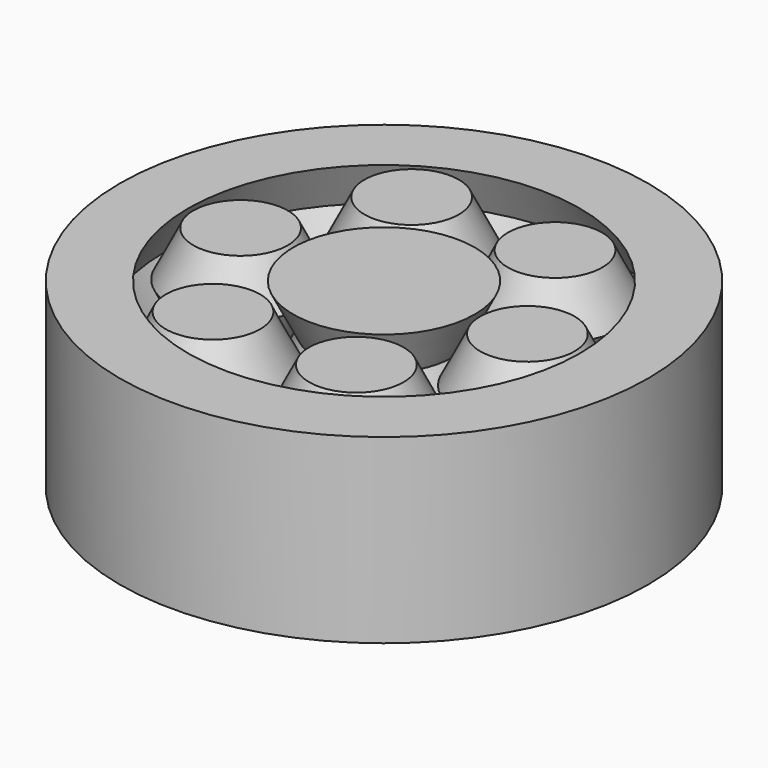
from build123d import *

# Parameters (mm, degrees)
F3_W     = 7.0104
F3_H     = 1.4224
F4_DEPTH = 1.905
F5_W     = 7.0104
F5_H     = 1.4224
F6_DEPTH = 1.905
F7_COUNT = 6


# Not quite as in the source:
# - a feature names something its author has since deleted; it is built from what else it names


with BuildPart() as f1:
    # F0 (on Front) → F1 (revolve)
    with BuildSketch(Plane.XZ):
        Polygon((8.4455, 12.7), (8.4455, 0), (10.033, 0), (11.6205, 0), (11.7475, 0), (13.335, 3.175), (13.081, 3.683), (11.7475, 6.35), (13.335, 9.525), (11.7475, 12.7), (11.6205, 12.7), (10.033, 12.7), align=None)
    revolve(axis=Axis((8.4455, 0, 6.35), (0, 0, -1)))

    # F5 (on face) → F6 (cut)
    with BuildSketch(Plane(origin=(0, 0, 0), x_dir=(1, 0, 0), z_dir=(0, 0, -1))):
        with Locations((8.4455, 0)):
            Rectangle(F5_W, F5_H)
    extrude(amount=-F6_DEPTH, mode=Mode.SUBTRACT)


with BuildPart() as f2:
    # F0 (on Front) → F2 (revolve)
    with BuildSketch(Plane.XZ):
        Polygon((-1.5875, 0), (0, 0), (3.175, 0), (4.7625, 0), (3.175, 3.175), (4.7625, 6.35), (3.175, 9.525), (4.7625, 12.7), (3.175, 12.7), (0, 12.7), (-1.5875, 12.7), align=None)
    revolve(axis=Axis((-1.5875, 0, 6.35), (0, 0, -1)))

    # F3 (on face) → F4 (cut)
    with BuildSketch(Plane(origin=(0, 0, 0), x_dir=(1, 0, 0), z_dir=(0, 0, -1))):
        with Locations((-1.5875, 0)):
            Rectangle(F3_W, F3_H)
    extrude(amount=-F4_DEPTH, mode=Mode.SUBTRACT)


with BuildPart() as f2b:
    # F0 (on Front) → F2, piece 2 (revolve)
    with BuildSketch(Plane.XZ):
        Polygon((13.716, 3.175), (12.1285, 0), (13.716, 0), (16.891, 0), (16.891, 12.7), (13.716, 12.7), (12.1285, 12.7), (13.716, 9.525), (12.1285, 6.35), align=None)
    revolve(axis=Axis((-1.5875, 0, 6.35), (0, 0, -1)))


with BuildPart() as f7_1:
    # F7: instance of F1
    add(f1.part.rotate(Axis((-1.5875, 0, 6.35), (0, 0, -1)), 1 * 360 / F7_COUNT))


with BuildPart() as f7_2:
    # F7: instance of F1
    add(f1.part.rotate(Axis((-1.5875, 0, 6.35), (0, 0, -1)), 2 * 360 / F7_COUNT))


with BuildPart() as f7_3:
    # F7: instance of F1
    add(f1.part.rotate(Axis((-1.5875, 0, 6.35), (0, 0, -1)), 3 * 360 / F7_COUNT))


with BuildPart() as f7_4:
    # F7: instance of F1
    add(f1.part.rotate(Axis((-1.5875, 0, 6.35), (0, 0, -1)), 4 * 360 / F7_COUNT))


with BuildPart() as f7_5:
    # F7: instance of F1
    add(f1.part.rotate(Axis((-1.5875, 0, 6.35), (0, 0, -1)), 5 * 360 / F7_COUNT))


solid = Compound([f1.part, f2.part, f2b.part, f7_1.part, f7_2.part, f7_3.part, f7_4.part, f7_5.part])
